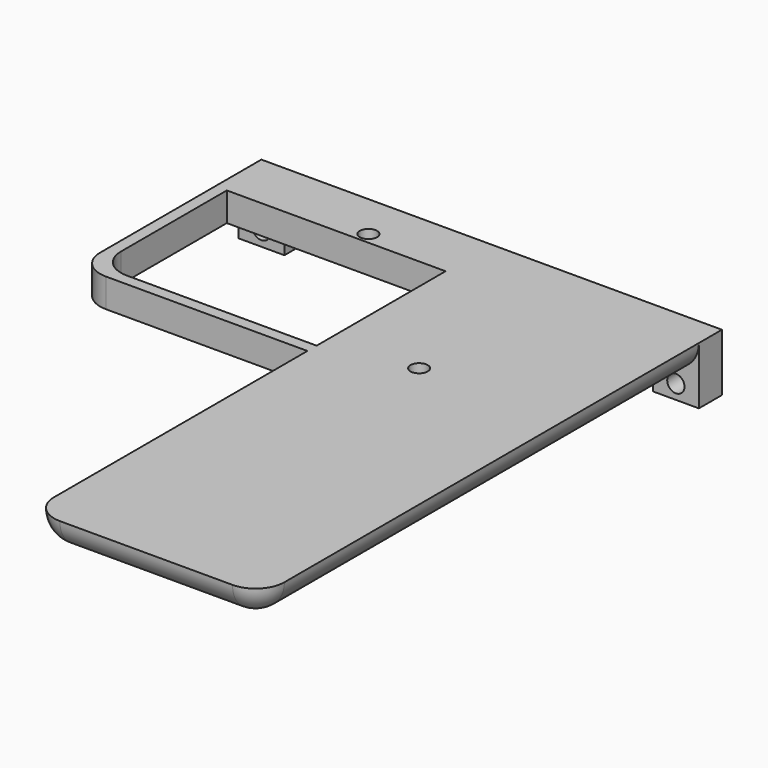
from build123d import *

# Parameters (mm, degrees)
F0_W     = 38
F0_H     = 10
F1_DEPTH = 5
F2_R     = 1.5
F3_DEPTH = 5
F4_W     = 8
F4_H     = 5
F5_DEPTH = 5
F6_R     = 1.5
F7_DEPTH = 5
F8_R     = 4.99999


# Not quite as in the source:
# - a fillet or chamfer is up to 0.001 mm smaller than in the source, because OpenCascade refuses the exact size
# - a feature names something its author has since deleted; it is built from what else it names


with BuildPart() as f1:
    # F0 (on Top) → F1 (new body)
    with BuildSketch(Plane.XY):
        Polygon((20, -50), (20, 50), (-20, 50), (-20, 40), (-20, 12), (-20, 10), (-20, -50), align=None)
        with Locations((-39, 45)):
            Rectangle(F0_W, F0_H)
        Polygon((-58, 40), (-58, 50), (-60, 50), (-60, 10), (-20, 10), (-20, 12), (-58, 12), align=None)
    extrude(amount=F1_DEPTH)

    # F2 (on face) → F3 (cut)
    with BuildSketch(Plane.XY.offset(5)):
        with Locations((-35, 42)):
            Circle(F2_R)
        with Locations((-5, 15.5)):
            Circle(F2_R)
    extrude(amount=-F3_DEPTH, mode=Mode.SUBTRACT)

    # F4 (on face) → F5 (join)
    with BuildSketch(Plane(origin=(0, 0, 0), x_dir=(1, 0, 0), z_dir=(0, 0, -1))):
        with Locations((16, -47.5)):
            Rectangle(F4_W, F4_H)
        with Locations((-56, -47.5)):
            Rectangle(F4_W, F4_H)
    extrude(amount=F5_DEPTH)

    # F6 (on face) → F7 (cut)
    with BuildSketch(Plane(origin=(0, 50, 0), x_dir=(-1, 0, 0), z_dir=(0, 1, 0))):
        with BuildLine():
            ThreePointArc((-14.5, -2.5), (-16, -1), (-17.5, -2.5))
            ThreePointArc((-17.5, -2.5), (-16, -4), (-14.5, -2.5))
        make_face()
        with Locations((56, -2.5)):
            Circle(F6_R)
    extrude(amount=-F7_DEPTH, mode=Mode.SUBTRACT)

    # F8 (radius 5 in the source; OpenCascade refuses exactly that, so slightly less here)
    f8_edges = [f1.edges().sort_by_distance(p)[0] for p in [
        (20, -2.5, 0),
        (-20, 26, 0),
        (-20, -20, 0),
        (20, -50, 2.5),
        (0, -50, 0),
        (-20, -50, 2.5),
        (-58, 12, 2.5),
        (-60, 10, 2.5),
    ]]
    fillet(f8_edges, radius=F8_R)


solid = f1.part
